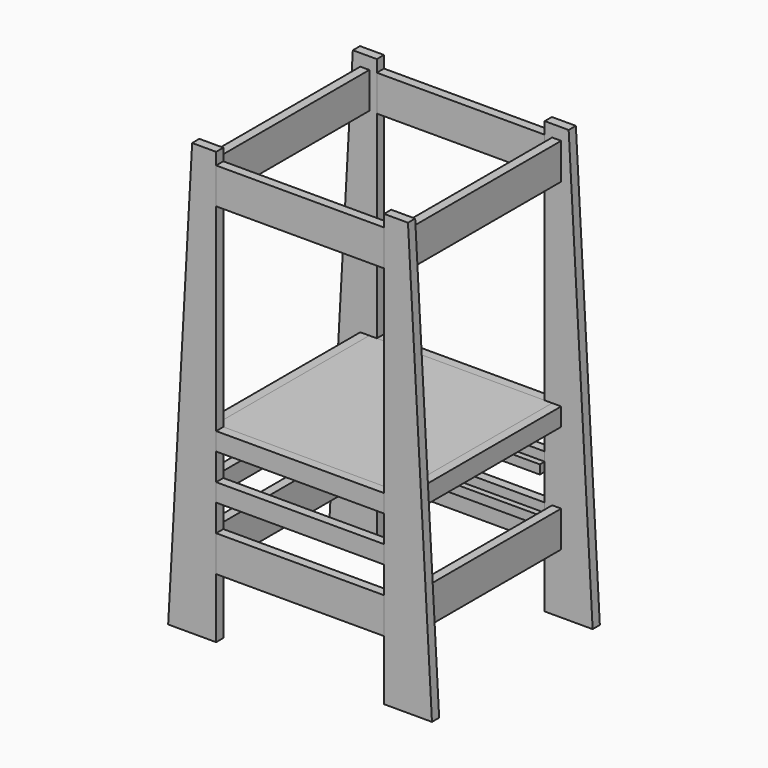
from build123d import *

# Parameters (mm, degrees)
F1_DEPTH       = 19.05
F0_W           = 355.6
F0_H           = 76.2
F2_DEPTH       = 19.05
F0_H_2         = 38.1
F4_DEPTH       = 12.7
F7_W           = 19.05
F7_H           = 76.2
F8_DEPTH       = 203.2
F8_DEPTH_BACK  = 203.2
F7_H_2         = 38.1
F9_W           = 387.35
F9_H           = 19.05
F10_DEPTH      = 203.2
F10_DEPTH_BACK = 203.2


with BuildPart() as f1:
    # F0 (on Front) → F1 (new body)
    with BuildSketch(Plane.XZ):
        Polygon((-228.6, 914.4), (-279.4, 0), (-177.8, 0), (-177.8, 127), (-177.8, 203.2), (-177.8, 260.35), (-177.8, 298.45), (-177.8, 355.6), (-177.8, 393.7), (-177.8, 812.8), (-177.8, 889), (-177.8, 914.4), align=None)
    extrude(amount=F1_DEPTH)


with BuildPart() as f1b:
    # F0 (on Front) → F1, piece 2 (new body)
    with BuildSketch(Plane.XZ):
        Polygon((177.8, 203.2), (177.8, 127), (177.8, 0), (279.4, 0), (228.6, 914.4), (177.8, 914.4), (177.8, 889), (177.8, 812.8), (177.8, 393.7), (177.8, 355.6), (177.8, 298.45), (177.8, 260.35), align=None)
    extrude(amount=F1_DEPTH)


with BuildPart() as f2:
    # F0 (on Front) → F2 (new body)
    with BuildSketch(Plane.XZ):
        with Locations((0, 850.9)):
            Rectangle(F0_W, F0_H)
    extrude(amount=F2_DEPTH)


with BuildPart() as f2b:
    # F0 (on Front) → F2, piece 2 (new body)
    with BuildSketch(Plane.XZ):
        with Locations((0, 374.65)):
            Rectangle(F0_W, F0_H_2)
    extrude(amount=F2_DEPTH)


with BuildPart() as f2c:
    # F0 (on Front) → F2, piece 3 (new body)
    with BuildSketch(Plane.XZ):
        with Locations((0, 279.4)):
            Rectangle(F0_W, F0_H_2)
    extrude(amount=F2_DEPTH)


with BuildPart() as f2d:
    # F0 (on Front) → F2, piece 4 (new body)
    with BuildSketch(Plane.XZ):
        with Locations((0, 165.1)):
            Rectangle(F0_W, F0_H)
    extrude(amount=F2_DEPTH)


with BuildPart() as f4:
    # F3 (on Front) → F4 (new body)
    with BuildSketch(Plane.XZ):
        Polygon((177.8, 355.6), (177.8, 374.65), (0, 374.65), (-177.8, 374.65), (-177.8, 355.6), (0, 355.6), align=None)
    extrude(amount=-F4_DEPTH)


with BuildPart() as f4b:
    # F3 (on Front) → F4, piece 2 (new body)
    with BuildSketch(Plane.XZ):
        Polygon((177.8, 260.35), (177.8, 279.4), (0, 279.4), (-177.8, 279.4), (-177.8, 260.35), (0, 260.35), align=None)
    extrude(amount=-F4_DEPTH)


with BuildPart() as f4c:
    # F3 (on Front) → F4, piece 3 (new body)
    with BuildSketch(Plane.XZ):
        Polygon((177.8, 165.1), (177.8, 184.15), (0, 184.15), (-177.8, 184.15), (-177.8, 165.1), (0, 165.1), align=None)
    extrude(amount=-F4_DEPTH)


with BuildPart() as f6_1:
    # F6: instance of F2
    add(f2.part.mirror(Plane.XZ.offset(-203.2)))


with BuildPart() as f6_2:
    # F6: instance of F2c
    add(f2c.part.mirror(Plane.XZ.offset(-203.2)))


with BuildPart() as f6_3:
    # F6: instance of F2d
    add(f2d.part.mirror(Plane.XZ.offset(-203.2)))


with BuildPart() as f6_4:
    # F6: instance of F4
    add(f4.part.mirror(Plane.XZ.offset(-203.2)))


with BuildPart() as f6_5:
    # F6: instance of F2b
    add(f2b.part.mirror(Plane.XZ.offset(-203.2)))


with BuildPart() as f6_6:
    # F6: instance of F1b
    add(f1b.part.mirror(Plane.XZ.offset(-203.2)))


with BuildPart() as f6_7:
    # F6: instance of F1
    add(f1.part.mirror(Plane.XZ.offset(-203.2)))


with BuildPart() as f6_8:
    # F6: instance of F4c
    add(f4c.part.mirror(Plane.XZ.offset(-203.2)))


with BuildPart() as f6_9:
    # F6: instance of F4b
    add(f4b.part.mirror(Plane.XZ.offset(-203.2)))


with BuildPart() as f8:
    # F7 (on offset) → F8 (new body, two sides)
    with BuildSketch(Plane.XZ.offset(-203.2)) as f8_sk:
        with Locations((203.2, 850.9)):
            Rectangle(F7_W, F7_H)
    extrude(amount=-F8_DEPTH)
    extrude(f8_sk.sketch, amount=F8_DEPTH_BACK)


with BuildPart() as f8b:
    # F7 (on offset) → F8, piece 2 (new body, two sides)
    with BuildSketch(Plane.XZ.offset(-203.2)) as f8_2_sk:
        with Locations((-203.2, 850.9)):
            Rectangle(F7_W, F7_H)
    extrude(amount=-F8_DEPTH)
    extrude(f8_2_sk.sketch, amount=F8_DEPTH_BACK)


with BuildPart() as f8c:
    # F7 (on offset) → F8, piece 3 (new body, two sides)
    with BuildSketch(Plane.XZ.offset(-203.2)) as f8_3_sk:
        with Locations((-203.2, 374.65)):
            Rectangle(F7_W, F7_H_2)
    extrude(amount=-F8_DEPTH)
    extrude(f8_3_sk.sketch, amount=F8_DEPTH_BACK)


with BuildPart() as f8d:
    # F7 (on offset) → F8, piece 4 (new body, two sides)
    with BuildSketch(Plane.XZ.offset(-203.2)) as f8_4_sk:
        with Locations((-203.2, 279.4)):
            Rectangle(F7_W, F7_H_2)
    extrude(amount=-F8_DEPTH)
    extrude(f8_4_sk.sketch, amount=F8_DEPTH_BACK)


with BuildPart() as f8e:
    # F7 (on offset) → F8, piece 5 (new body, two sides)
    with BuildSketch(Plane.XZ.offset(-203.2)) as f8_5_sk:
        with Locations((-203.2, 165.1)):
            Rectangle(F7_W, F7_H)
    extrude(amount=-F8_DEPTH)
    extrude(f8_5_sk.sketch, amount=F8_DEPTH_BACK)


with BuildPart() as f8f:
    # F7 (on offset) → F8, piece 6 (new body, two sides)
    with BuildSketch(Plane.XZ.offset(-203.2)) as f8_6_sk:
        with Locations((203.2, 165.1)):
            Rectangle(F7_W, F7_H)
    extrude(amount=-F8_DEPTH)
    extrude(f8_6_sk.sketch, amount=F8_DEPTH_BACK)


with BuildPart() as f8g:
    # F7 (on offset) → F8, piece 7 (new body, two sides)
    with BuildSketch(Plane.XZ.offset(-203.2)) as f8_7_sk:
        with Locations((203.2, 374.65)):
            Rectangle(F7_W, F7_H_2)
    extrude(amount=-F8_DEPTH)
    extrude(f8_7_sk.sketch, amount=F8_DEPTH_BACK)


with BuildPart() as f10:
    # F9 (on offset) → F10 (new body, two sides)
    with BuildSketch(Plane.XZ.offset(-203.2)) as f10_sk:
        with Locations((0, 384.175)):
            Rectangle(F9_W, F9_H)
    extrude(amount=-F10_DEPTH)
    extrude(f10_sk.sketch, amount=F10_DEPTH_BACK)


solid = Compound([f1.part, f1b.part, f2.part, f2b.part, f2c.part, f2d.part, f4.part, f4b.part, f4c.part, f6_1.part, f6_2.part, f6_3.part, f6_4.part, f6_5.part, f6_6.part, f6_7.part, f6_8.part, f6_9.part, f8.part, f8b.part, f8c.part, f8d.part, f8e.part, f8f.part, f8g.part, f10.part])
